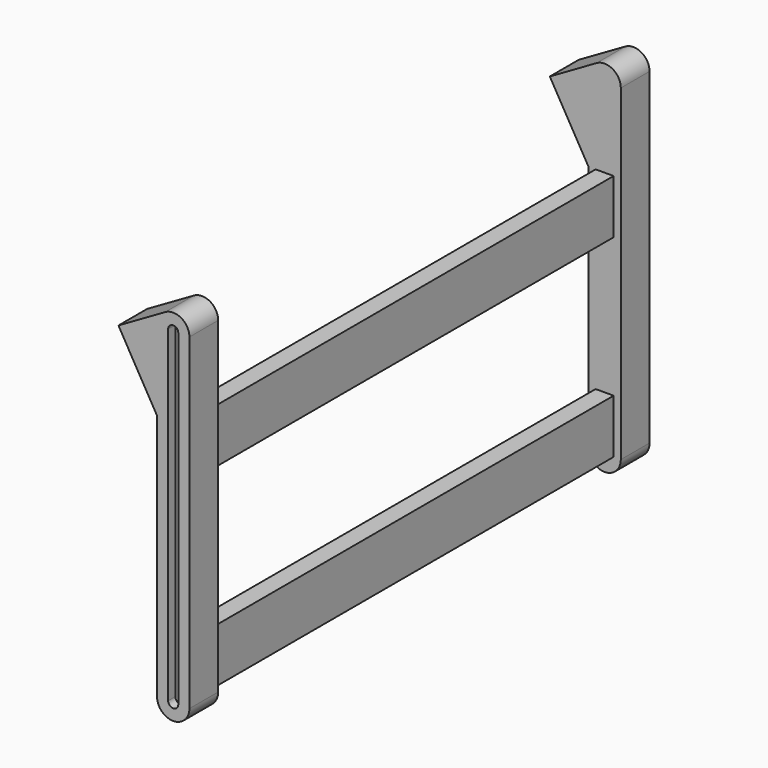
from build123d import *

# Parameters (mm, degrees)
F1_DEPTH      = 25.4
F2_START      = -381
F2_DEPTH      = 25.4
F3_W          = 12.7
F3_H          = 38.1
F4_DEPTH      = 361.95
F4_DEPTH_BACK = 6.35
F6_DEPTH      = 6.35
F7_START      = -400.05
F7_DEPTH      = 6.35


# Not quite as in the source:
# - a feature of the source that left no trace in its solid (it failed there, or was rolled back) is left out


with BuildPart() as f1:
    # F0 (on Front) → F1 (new body)
    with BuildSketch(Plane.XZ):
        with BuildLine():
            Line((-11.43, 174.7373407305), (-11.43, 0))
            ThreePointArc((-11.43, 0), (0, -11.43), (11.43, 0))
            Line((11.43, 0), (11.43, 231.14))
            ThreePointArc((11.43, 231.14), (5.715, 241.0386703653), (-5.715, 241.0386703653))
            Line((-5.715, 241.0386703653), (-38.7105678842, 221.9886703653))
            Line((-38.7105678842, 221.9886703653), (-11.43, 174.7373407305))
        make_face()
        with BuildLine():
            Line((-3.571875, 0), (-3.571875, 231.14))
            ThreePointArc((-3.571875, 231.14), (0, 234.711875), (3.571875, 231.14))
            Line((3.571875, 231.14), (3.571875, 0))
            ThreePointArc((3.571875, 0), (0, -3.571875), (-3.571875, 0))
        make_face(mode=Mode.SUBTRACT)
        with BuildLine():
            ThreePointArc((3.571875, 231.14), (0, 234.711875), (-3.571875, 231.14))
            Line((-3.571875, 231.14), (-3.571875, 0))
            ThreePointArc((-3.571875, 0), (0, -3.571875), (3.571875, 0))
            Line((3.571875, 0), (3.571875, 231.14))
        make_face()
    extrude(amount=-F1_DEPTH)



with BuildPart() as f2:
    # F0 (on Front) → F2 (new body)
    with BuildSketch(Plane.XZ.offset(F2_START)):
        with BuildLine():
            Line((-11.43, 174.7373407305), (-11.43, 0))
            ThreePointArc((-11.43, 0), (0, -11.43), (11.43, 0))
            Line((11.43, 0), (11.43, 231.14))
            ThreePointArc((11.43, 231.14), (5.715, 241.0386703653), (-5.715, 241.0386703653))
            Line((-5.715, 241.0386703653), (-38.7105678842, 221.9886703653))
            Line((-38.7105678842, 221.9886703653), (-11.43, 174.7373407305))
        make_face()
        with BuildLine():
            Line((-3.571875, 0), (-3.571875, 231.14))
            ThreePointArc((-3.571875, 231.14), (0, 234.711875), (3.571875, 231.14))
            Line((3.571875, 231.14), (3.571875, 0))
            ThreePointArc((3.571875, 0), (0, -3.571875), (-3.571875, 0))
        make_face(mode=Mode.SUBTRACT)
        with BuildLine():
            ThreePointArc((3.571875, 231.14), (0, 234.711875), (-3.571875, 231.14))
            Line((-3.571875, 231.14), (-3.571875, 0))
            ThreePointArc((-3.571875, 0), (0, -3.571875), (3.571875, 0))
            Line((3.571875, 0), (3.571875, 231.14))
        make_face()
    extrude(amount=-F2_DEPTH)


with BuildPart() as f1_1:
    add(f1.part)

    add(f2.part)  # F4 merges F2
    # F3 (on face) → F4 (join, two sides)
    with BuildSketch(Plane(origin=(0, 25.4, 0), x_dir=(-1, 0, 0), z_dir=(0, 1, 0))) as f4_sk:
        with Locations((0, 155.6873407305)):
            Rectangle(F3_W, F3_H)
        with Locations((0, 19.05)):
            Rectangle(F3_W, F3_H)
    extrude(amount=F4_DEPTH)
    extrude(f4_sk.sketch, amount=-F4_DEPTH_BACK)

    # F0 (on Front) → F6 (cut)
    with BuildSketch(Plane.XZ):
        with BuildLine():
            ThreePointArc((3.571875, 231.14), (0, 234.711875), (-3.571875, 231.14))
            Line((-3.571875, 231.14), (-3.571875, 0))
            ThreePointArc((-3.571875, 0), (0, -3.571875), (3.571875, 0))
            Line((3.571875, 0), (3.571875, 231.14))
        make_face()
    extrude(amount=-F6_DEPTH, mode=Mode.SUBTRACT)

    # F0 (on Front) → F7 (cut)
    with BuildSketch(Plane.XZ.offset(F7_START)):
        with BuildLine():
            ThreePointArc((3.571875, 231.14), (0, 234.711875), (-3.571875, 231.14))
            Line((-3.571875, 231.14), (-3.571875, 0))
            ThreePointArc((-3.571875, 0), (0, -3.571875), (3.571875, 0))
            Line((3.571875, 0), (3.571875, 231.14))
        make_face()
    extrude(amount=-F7_DEPTH, mode=Mode.SUBTRACT)


solid = f1_1.part
